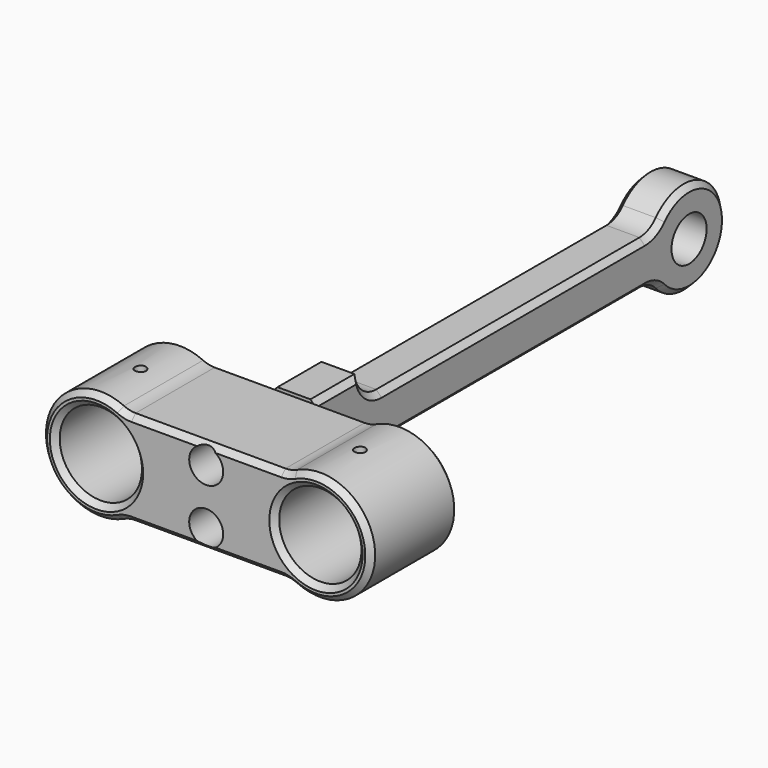
from build123d import *

# Parameters (mm, degrees)
F0_R          = 7.5
F0_R_2        = 1.6
F1_DEPTH      = 20
F2_W          = 8
F2_H          = 17
F2_R          = 1.1
F3_DEPTH      = 95
F4_DEPTH      = 7
F5_R          = 3.1
F5_R_2        = 1.6
F6_DEPTH      = 10
F7_R          = 4
F8_DEPTH      = 25
F12_DEPTH     = 15
F14_R         = 5
F15_R         = 5
F16_DEPTH     = 12.5
F17_T1_DEPTH  = 8
F18_R         = 5
F19_T1_DEPTH  = 27.3216296593
F19_T12_ANGLE = 24.9996259311
F19_T14_ANGLE = 24.9996259311
F19_T16_ANGLE = 229.9992518621
F19_T18_ANGLE = 24.9996259311
F19_T20_ANGLE = 24.9996259311
F19_T22_ANGLE = 229.9992518621
F19_T24_ANGLE = 24.9996259311
F19_T26_ANGLE = 24.9996259311
F19_T28_ANGLE = 229.9992518621
F19_T30_ANGLE = 24.9996259311
F19_T32_ANGLE = 24.9996259311
F19_T34_ANGLE = 229.9992518621
F20_SIZE      = 1


# Not quite as in the source:
# - a fillet or chamfer that OpenCascade refuses, or shapes differently, is made with other operations: its cross-section is extruded or revolved along the edge and cut away or added
# - a feature names something its author has since deleted; it is built from what else it names


with BuildPart() as f1:
    # F0 (on Front) → F1 (new body)
    with BuildSketch(Plane.XZ):
        with BuildLine():
            Line((14.8880678261, 8.5946581927), (-14.8880678261, 8.5946581927))
            ThreePointArc((-14.8880678261, 8.5946581927), (-30, 0), (-14.8880678261, -8.5946581927))
            Line((-14.8880678261, -8.5946581927), (14.8880678261, -8.5946581927))
            ThreePointArc((14.8880678261, -8.5946581927), (30, 0), (14.8880678261, 8.5946581927))
        make_face()
        with Locations((-20, 0)):
            Circle(F0_R, mode=Mode.SUBTRACT)
        with Locations((0, -5)):
            Circle(F0_R_2, mode=Mode.SUBTRACT)
        with Locations((20, 0)):
            Circle(F0_R, mode=Mode.SUBTRACT)
        with Locations((0, 5)):
            Circle(F0_R_2, mode=Mode.SUBTRACT)
    extrude(amount=F1_DEPTH)

    # F5 (on face) → F6 (cut)
    with BuildSketch(Plane.XZ.offset(20)):
        with Locations((0, 5)):
            Circle(F5_R)
        with Locations((0, 5)):
            Circle(F5_R_2, mode=Mode.SUBTRACT)
        with Locations((0, -5)):
            Circle(F5_R)
        with Locations((0, -5)):
            Circle(F5_R_2, mode=Mode.SUBTRACT)
    extrude(amount=-F6_DEPTH, mode=Mode.SUBTRACT)

    # F11 (on Top) → F12 (cut)
    with BuildSketch(Plane.XY):
        with BuildLine():
            ThreePointArc((-19, -10), (-20, -9), (-21, -10))
            Line((-21, -10), (-19, -10))
        make_face()
        with BuildLine():
            ThreePointArc((21, -10), (20, -9), (19, -10))
            Line((19, -10), (21, -10))
        make_face()
        with BuildLine():
            Line((21, -10), (19, -10))
            ThreePointArc((19, -10), (20, -11), (21, -10))
        make_face()
        with BuildLine():
            Line((-19, -10), (-21, -10))
            ThreePointArc((-21, -10), (-20, -11), (-19, -10))
        make_face()
    extrude(amount=F12_DEPTH, mode=Mode.SUBTRACT)

    # F14
    f14_edges = [f1.edges().sort_by_distance(p)[0] for p in [
        (-14.888068, -10, 8.594658),
    ]]
    fillet(f14_edges, radius=F14_R)

    # F15
    f15_edges = [f1.edges().sort_by_distance(p)[0] for p in [
        (-14.888068, -10, -8.594658),
        (14.888068, -10, -8.594658),
        (14.888068, -10, 8.594658),
    ]]
    fillet(f15_edges, radius=F15_R)

    # F19: chamfer of 1 on 6 edges, made by hand

    # F19_s2 → F19_t1 (cut)
    with BuildSketch(Plane.YZ.offset(-13.6608148297)):
        Polygon((0, -7.5946581927), (-1, -8.5946581927), (0, -8.5946581927), align=None)
        Polygon((-19, -8.5946581927), (-20, -7.5946581927), (-20, -8.5946581927), align=None)
        Polygon((-19, 8.5946581927), (-20, 7.5946581927), (-20, 8.5946581927), align=None)
        Polygon((0, 7.5946581927), (-1, 8.5946581927), (0, 8.5946581927), align=None)
    extrude(amount=F19_T1_DEPTH, mode=Mode.SUBTRACT)

    # F19_s3 → F19_t4 (revolve, cut)
    with BuildSketch(Plane.XY):
        Polygon((-11.5, 0), (-12.5, -1), (-12.5, 0), align=None)
    revolve(axis=Axis((-20, 0, 0), (0, -1, 0)), mode=Mode.SUBTRACT)

    # F19_s5 → F19_t6 (revolve, cut)
    with BuildSketch(Plane.XY):
        Polygon((28.5, 0), (27.5, -1), (27.5, 0), align=None)
    revolve(axis=Axis((20, 0, 0), (0, -1, 0)), mode=Mode.SUBTRACT)

    # F19_s7 → F19_t8 (revolve, cut)
    with BuildSketch(Plane.XY):
        Polygon((-12.5, -19), (-11.5, -20), (-12.5, -20), align=None)
    revolve(axis=Axis((-20, -20, 0), (0, -1, 0)), mode=Mode.SUBTRACT)

    # F19_s9 → F19_t10 (revolve, cut)
    with BuildSketch(Plane.XY):
        Polygon((27.5, -19), (28.5, -20), (27.5, -20), align=None)
    revolve(axis=Axis((20, -20, 0), (0, -1, 0)), mode=Mode.SUBTRACT)

    # F19_s11 → F19_t12 (revolve, cut)
    with BuildSketch(Plane(origin=(-16.4279761223, 0, -7.6603604987), x_dir=(0, 1, 0), z_dir=(-0.9063105462, 0, -0.4226123447))):
        Polygon((-19, 1.5477531062), (-20, 0.5477531062), (-20, 1.5477531062), align=None)
    revolve(axis=Axis((-13.6608148297, -20, -13.5946581927), (0, 1, 0)), revolution_arc=F19_T12_ANGLE, mode=Mode.SUBTRACT)

    # F19_s13 → F19_t14 (revolve, cut)
    with BuildSketch(Plane(origin=(16.4279761223, 0, -7.6603604987), x_dir=(0, 1, 0), z_dir=(0.9063105462, 0, -0.4226123447))):
        Polygon((-19, -1.5477531062), (-20, -0.5477531062), (-20, -1.5477531062), align=None)
    revolve(axis=Axis((13.6608148297, -20, -13.5946581927), (0, -1, 0)), revolution_arc=F19_T14_ANGLE, mode=Mode.SUBTRACT)

    # F19_s15 → F19_t16 (revolve, cut)
    with BuildSketch(Plane(origin=(16.4279761223, 0, -7.6603604987), x_dir=(0, 1, 0), z_dir=(-0.9063105462, 0, 0.4226123447))):
        Polygon((-19, 1.5477531062), (-20, 0.5477531062), (-20, 1.5477531062), align=None)
    revolve(axis=Axis((20, -20, 0), (0, -1, 0)), revolution_arc=F19_T16_ANGLE, mode=Mode.SUBTRACT)

    # F19_s17 → F19_t18 (revolve, cut)
    with BuildSketch(Plane.YZ.offset(13.6608148297)):
        Polygon((-19, 8.5946581927), (-20, 7.5946581927), (-20, 8.5946581927), align=None)
    revolve(axis=Axis((13.6608148297, -20, 13.5946581927), (0, -1, 0)), revolution_arc=F19_T18_ANGLE, mode=Mode.SUBTRACT)

    # F19_s19 → F19_t20 (revolve, cut)
    with BuildSketch(Plane.YZ.offset(-13.6608148297)):
        Polygon((-19, 8.5946581927), (-20, 7.5946581927), (-20, 8.5946581927), align=None)
    revolve(axis=Axis((-13.6608148297, -20, 13.5946581927), (0, 1, 0)), revolution_arc=F19_T20_ANGLE, mode=Mode.SUBTRACT)

    # F19_s21 → F19_t22 (revolve, cut)
    with BuildSketch(Plane(origin=(-16.4279761223, 0, 7.6603604987), x_dir=(0, 1, 0), z_dir=(0.9063105462, 0, -0.4226123447))):
        Polygon((-19, 1.5477531062), (-20, 0.5477531062), (-20, 1.5477531062), align=None)
    revolve(axis=Axis((-20, -20, 0), (0, -1, 0)), revolution_arc=F19_T22_ANGLE, mode=Mode.SUBTRACT)

    # F19_s23 → F19_t24 (revolve, cut)
    with BuildSketch(Plane(origin=(-16.4279761223, 0, -7.6603604987), x_dir=(0, 1, 0), z_dir=(-0.9063105462, 0, -0.4226123447))):
        Polygon((0, 0.5477531062), (-1, 1.5477531062), (0, 1.5477531062), align=None)
    revolve(axis=Axis((-13.6608148297, 0, -13.5946581927), (0, 1, 0)), revolution_arc=F19_T24_ANGLE, mode=Mode.SUBTRACT)

    # F19_s25 → F19_t26 (revolve, cut)
    with BuildSketch(Plane(origin=(16.4279761223, 0, -7.6603604987), x_dir=(0, 1, 0), z_dir=(0.9063105462, 0, -0.4226123447))):
        Polygon((0, -0.5477531062), (-1, -1.5477531062), (0, -1.5477531062), align=None)
    revolve(axis=Axis((13.6608148297, 0, -13.5946581927), (0, -1, 0)), revolution_arc=F19_T26_ANGLE, mode=Mode.SUBTRACT)

    # F19_s27 → F19_t28 (revolve, cut)
    with BuildSketch(Plane(origin=(16.4279761223, 0, -7.6603604987), x_dir=(0, 1, 0), z_dir=(-0.9063105462, 0, 0.4226123447))):
        Polygon((0, 0.5477531062), (-1, 1.5477531062), (0, 1.5477531062), align=None)
    revolve(axis=Axis((20, 0, 0), (0, -1, 0)), revolution_arc=F19_T28_ANGLE, mode=Mode.SUBTRACT)

    # F19_s29 → F19_t30 (revolve, cut)
    with BuildSketch(Plane.YZ.offset(13.6608148297)):
        Polygon((0, 7.5946581927), (-1, 8.5946581927), (0, 8.5946581927), align=None)
    revolve(axis=Axis((13.6608148297, 0, 13.5946581927), (0, -1, 0)), revolution_arc=F19_T30_ANGLE, mode=Mode.SUBTRACT)

    # F19_s31 → F19_t32 (revolve, cut)
    with BuildSketch(Plane.YZ.offset(-13.6608148297)):
        Polygon((0, 7.5946581927), (-1, 8.5946581927), (0, 8.5946581927), align=None)
    revolve(axis=Axis((-13.6608148297, 0, 13.5946581927), (0, 1, 0)), revolution_arc=F19_T32_ANGLE, mode=Mode.SUBTRACT)

    # F19_s33 → F19_t34 (revolve, cut)
    with BuildSketch(Plane(origin=(-16.4279761223, 0, 7.6603604987), x_dir=(0, 1, 0), z_dir=(0.9063105462, 0, -0.4226123447))):
        Polygon((0, 0.5477531062), (-1, 1.5477531062), (0, 1.5477531062), align=None)
    revolve(axis=Axis((-20, 0, 0), (0, -1, 0)), revolution_arc=F19_T34_ANGLE, mode=Mode.SUBTRACT)


with BuildPart() as f3:
    # F2 (on face) → F3 (new body)
    with BuildSketch(Plane(origin=(0, 0, 0), x_dir=(-1, 0, 0), z_dir=(0, 1, 0))):
        Rectangle(F2_W, F2_H)
        with Locations((0, -5)):
            Circle(F2_R, mode=Mode.SUBTRACT)
        with Locations((0, 5)):
            Circle(F2_R, mode=Mode.SUBTRACT)
        with Locations((0, 5)):
            Circle(F2_R)
        with Locations((0, -5)):
            Circle(F2_R)
    extrude(amount=F3_DEPTH)

    # F2 (on face) → F4 (cut)
    with BuildSketch(Plane(origin=(0, 0, 0), x_dir=(-1, 0, 0), z_dir=(0, 1, 0))):
        with Locations((0, 5)):
            Circle(F2_R)
        with Locations((0, -5)):
            Circle(F2_R)
    extrude(amount=F4_DEPTH, mode=Mode.SUBTRACT)

    # F7 (on face) → F8 (cut)
    with BuildSketch(Plane(origin=(-4, 0, 0), x_dir=(0, -1, 0), z_dir=(-1, 0, 0))):
        with Locations((-85, 0)):
            Circle(F7_R)
    extrude(amount=-F8_DEPTH, mode=Mode.SUBTRACT)

    # F13 (on Right) → F16 (cut, symmetric)
    with BuildSketch(Plane.YZ):
        with BuildLine():
            ThreePointArc((77.5, 4), (93.5, 0), (77.5, -4))
            Line((77.5, -4), (10, -4))
            Line((10, -4), (10, -10))
            Line((10, -10), (0, -10))
            Line((0, -10), (0, -17.4690615386))
            Line((0, -17.4690615386), (98.2531383634, -15.3523003682))
            Line((98.2531383634, -15.3523003682), (98.2531383634, 24.7300937772))
            Line((98.2531383634, 24.7300937772), (0, 24.7300937772))
            Line((0, 24.7300937772), (0, 10))
            Line((0, 10), (10, 10))
            Line((10, 10), (10, 4))
            Line((10, 4), (77.5, 4))
        make_face()
    extrude(amount=F16_DEPTH, both=True, mode=Mode.SUBTRACT)

    # F17: fillet of radius 5 on 2 edges, made by hand

    # F17_s2 → F17_t1 (join)
    with BuildSketch(Plane.YZ.offset(-4)):
        with BuildLine():
            ThreePointArc((14.9749371855, 4), (11.6208352193, 5.2919007565), (10, 8.5))
            Line((10, 8.5), (10, 4))
            Line((10, 4), (14.9749371855, 4))
        make_face()
        with BuildLine():
            ThreePointArc((14.9749371855, -4), (11.6208352193, -5.2919007565), (10, -8.5))
            Line((10, -8.5), (10, -4))
            Line((10, -4), (14.9749371855, -4))
        make_face()
    extrude(amount=F17_T1_DEPTH)

    # F18
    f18_edges = [f3.edges().sort_by_distance(p)[0] for p in [
        (0, 77.5, 4),
        (0, 77.5, -4),
    ]]
    fillet(f18_edges, radius=F18_R)

    # F20
    f20_edges = [f3.edges().sort_by_distance(p)[0] for p in [
        (4, 44.956316, -4),
        (-4, 44.956316, -4),
        (4, 5, -8.5),
        (4, 5, 8.5),
        (-4, 5, -8.5),
        (-4, 5, 8.5),
        (-4, 76.978936, -4.435645),
        (-4, 11.620835, -5.291901),
        (-4, 93.5, 0),
        (-4, 76.978936, 4.435645),
        (-4, 44.956316, 4),
        (-4, 11.620835, 5.291901),
        (4, 76.978936, -4.435645),
        (4, 11.620835, -5.291901),
        (4, 93.5, 0),
        (4, 76.978936, 4.435645),
        (4, 44.956316, 4),
        (4, 11.620835, 5.291901),
    ]]
    chamfer(f20_edges, length=F20_SIZE)


solid = Compound([f1.part, f3.part])
